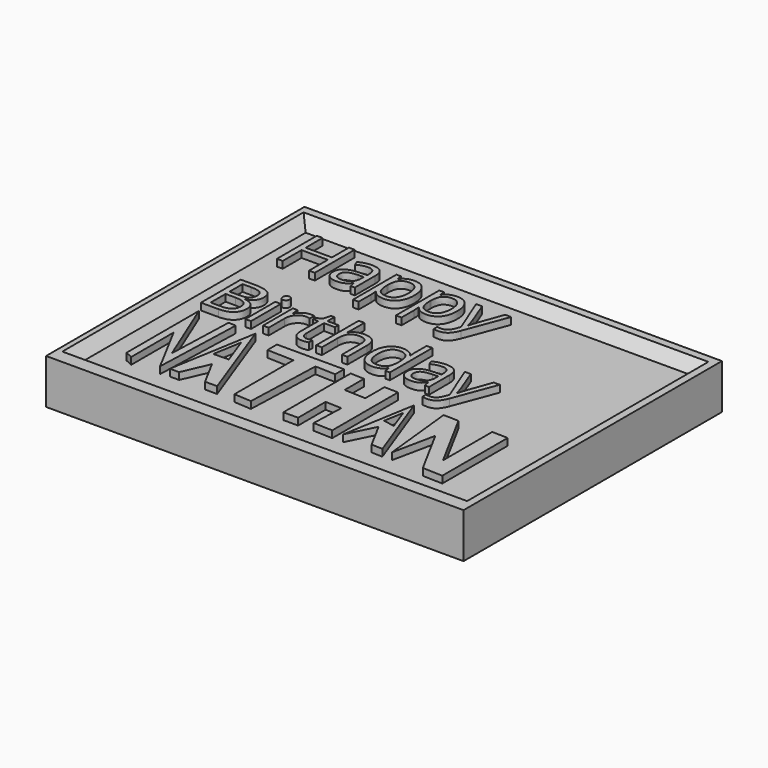
from build123d import *

# Parameters (mm, degrees)
F1_W         = 153.5131447017
F1_H         = 118.7682263553
F1_W_2       = 138.6890634894
F1_H_2       = 100.725505501
F2_DEPTH     = 16.51
F3_DEPTH     = 12.7
F0_TEXT_SIZE = 25.6912866866
F4_DEPTH     = 15.24
F5_T4_DEPTH  = 138.6890634894
F5_T9_DEPTH  = 100.725505501
F5_T14_DEPTH = 138.6890634894
F5_T19_DEPTH = 100.725505501
F5_T25_DEPTH = 113.7896550799
F5_T30_DEPTH = 151.7532130683
F5_T38_DEPTH = 151.7532130683
F5_T43_DEPTH = 113.7896550799
F5_T51_DEPTH = 113.7896550799
F5_T56_DEPTH = 151.7532130683
F5_T64_DEPTH = 113.7896550799
F5_T69_DEPTH = 151.7532130683


# Not quite as in the source:
# - a fillet or chamfer that OpenCascade refuses, or shapes differently, is made with other operations: its cross-section is extruded or revolved along the edge and cut away or added
# - Text() gives the source's letters only with a copy of the font that has no kerning and outlines rounded to 1/6400 em; it was checked with that copy


with BuildPart() as f2:
    # F1 (on Top) → F2 (new body)
    with BuildSketch(Plane.XY):
        with Locations((-23.7906444818, -12.9123348743)):
            Rectangle(F1_W, F1_H)
        with Locations((-24.1845287383, -11.8035394698)):
            Rectangle(F1_W_2, F1_H_2, mode=Mode.SUBTRACT)
    extrude(amount=F2_DEPTH)

    # F1 (on Top) → F3 (join)
    with BuildSketch(Plane.XY):
        with Locations((-24.1845287383, -11.8035394698)):
            Rectangle(F1_W_2, F1_H_2)
    extrude(amount=F3_DEPTH)

    # F0 (on Top) → F4 (join)
    with BuildSketch(Plane.XY):
        Polygon((-85.3031873703, -21.0467930883), (-85.3031873703, -54.3782301247), (-82.5872942805, -55.6127279997), (-82.5872942805, -36.1076667905), (-72.49553914, -54.9944023292), (-71.3395271598, -21.6351880797), (-74.0692615509, -21.5405933559), (-74.9334096909, -46.4774481952), align=None)
        Polygon((-63.8229250908, -22.0343936235), (-69.3781673908, -54.3782301247), (-65.9531280398, -54.3782301247), (-61.6957172751, -44.6236543357), (-56.4159415662, -54.3782301247), (-51.9717484713, -54.3782301247), align=None)
        Polygon((-59.7228327978, -39.3131503296), (-65.3510764241, -39.4346043468), (-63.5406248941, -28.8937593002), align=None, mode=Mode.SUBTRACT)
        Polygon((-44.9698902667, -28.1148646027), (-44.9698902667, -55.175434798), (-38.6008597223, -55.5698666259), (-37.6162595271, -27.157108435), (-30.1302243024, -27.4165254086), (-30.1302243024, -23.4010890126), (-54.7469718501, -23.4010890126), (-54.7469718501, -27.7760549605), align=None)
        Polygon((-26.9877053797, -24.2740083486), (-26.9877053797, -55.175434798), (-21.5674239871, -55.175434798), (-21.5674239871, -42.544283495), (-15.5946510085, -42.7512607057), (-16.0167792908, -54.9326810121), (-9.0115962201, -55.175434798), (-9.0115962201, -24.9731168782), (-14.0718441197, -24.7977618128), (-14.0718441197, -33.6245252917), (-21.92478826, -33.352393657), (-21.92478826, -24.4494559116), align=None)
        Polygon((-0.3970701119, -28.3770595024), (-4.9998471513, -55.175434798), (0, -45.1317872426), (5.3600473669, -55.0346678109), (9.4221818105, -55.175434798), align=None)
        Polygon((3.0691473118, -41.9747008738), (-1.1165549513, -41.2297546864), (0.1321939148, -33.9592654843), align=None, mode=Mode.SUBTRACT)
        Polygon((10.0144669414, -27.7569666505), (12.9211032763, -55.175434798), (16.226188811, -39.3131503296), (25.9121123405, -57.2082429175), (33.2773711625, -57.4634745717), (33.2773711625, -27.4220021975), (27.4817449731, -27.2211637348), (27.4817449731, -49.8912126499), (15.6062132016, -27.9507399696), align=None)
        with Locations((-90.5801325571, 18.2041097432)):
            Text('Happy', F0_TEXT_SIZE, font='Open Sans', text_align=(TextAlign.LEFT, TextAlign.BOTTOM))
        with Locations((-90.5801325571, -16.7360401505)):
            Text('Birthday', F0_TEXT_SIZE, font='Open Sans', text_align=(TextAlign.LEFT, TextAlign.BOTTOM))
    extrude(amount=F4_DEPTH)

    # F5: chamfer of 5.08 on 4 edges, made by hand


with BuildPart() as f5_tool2:
    # F5_s3 → F5_t4 (new body)
    with BuildSketch(Plane.YZ.offset(-93.529060483)):
        Polygon((43.6392132807, 16.51), (38.5592132807, 11.43), (38.5592132807, 16.51), align=None)
    extrude(amount=F5_T4_DEPTH)

    split(bisect_by=Plane.XY.offset(12.7), keep=Keep.TOP)


with BuildPart() as f2_1:
    add(f2.part)

    # F5_t1: cut F5_tool2
    add(f5_tool2.part, mode=Mode.SUBTRACT)


with BuildPart() as f5_tool7:
    # F5_s8 → F5_t9 (new body)
    with BuildSketch(Plane.XZ.offset(-38.5592132807)):
        Polygon((50.2400030065, 16.51), (45.1600030065, 11.43), (45.1600030065, 16.51), align=None)
    extrude(amount=F5_T9_DEPTH)

    split(bisect_by=Plane.XY.offset(12.7), keep=Keep.TOP)


with BuildPart() as f2_2:
    add(f2_1.part)

    # F5_t6: cut F5_tool7
    add(f5_tool7.part, mode=Mode.SUBTRACT)


with BuildPart() as f5_tool12:
    # F5_s13 → F5_t14 (new body)
    with BuildSketch(Plane.YZ.offset(45.1600030065)):
        Polygon((-67.2462922204, 16.51), (-62.1662922204, 11.43), (-62.1662922204, 16.51), align=None)
    extrude(amount=-F5_T14_DEPTH)

    split(bisect_by=Plane.XY.offset(12.7), keep=Keep.TOP)


with BuildPart() as f2_3:
    add(f2_2.part)

    # F5_t11: cut F5_tool12
    add(f5_tool12.part, mode=Mode.SUBTRACT)


with BuildPart() as f5_tool17:
    # F5_s18 → F5_t19 (new body)
    with BuildSketch(Plane.XZ.offset(62.1662922204)):
        Polygon((-98.609060483, 16.51), (-93.529060483, 11.43), (-93.529060483, 16.51), align=None)
    extrude(amount=-F5_T19_DEPTH)

    split(bisect_by=Plane.XY.offset(12.7), keep=Keep.TOP)


with BuildPart() as f2_4:
    add(f2_3.part)

    # F5_t16: cut F5_tool17
    add(f5_tool17.part, mode=Mode.SUBTRACT)


with BuildPart() as f5_tool23:
    # F5_s24 → F5_t25 (new body)
    with BuildSketch(Plane.XZ.offset(62.1662922204)):
        Polygon((-98.609060483, 16.51), (-93.529060483, 11.43), (-93.529060483, 16.51), align=None)
    extrude(amount=-F5_T25_DEPTH)

    split(bisect_by=Plane.XY.offset(12.7), keep=Keep.TOP)

    split(bisect_by=Plane.XZ.offset(-38.5592132807), keep=Keep.BOTTOM)


with BuildPart() as f5_tool28:
    # F5_s29 → F5_t30 (new body)
    with BuildSketch(Plane.YZ.offset(-106.5932100618)):
        Polygon((43.6392132807, 16.51), (38.5592132807, 11.43), (38.5592132807, 16.51), align=None)
    extrude(amount=F5_T30_DEPTH)

    split(bisect_by=Plane.YZ.offset(-93.529060483), keep=Keep.BOTTOM)

    split(bisect_by=Plane.XY.offset(12.7), keep=Keep.TOP)


with BuildPart() as f5_tool23_1:
    add(f5_tool23.part)

    # F5_t33: intersect F5_tool28
    add(f5_tool28.part, mode=Mode.INTERSECT)


with BuildPart() as f2_5:
    add(f2_4.part)

    # F5_t21: cut F5_tool23
    add(f5_tool23_1.part, mode=Mode.SUBTRACT)


with BuildPart() as f5_tool36:
    # F5_s37 → F5_t38 (new body)
    with BuildSketch(Plane.YZ.offset(-93.529060483)):
        Polygon((43.6392132807, 16.51), (38.5592132807, 11.43), (38.5592132807, 16.51), align=None)
    extrude(amount=F5_T38_DEPTH)

    split(bisect_by=Plane.XY.offset(12.7), keep=Keep.TOP)

    split(bisect_by=Plane.YZ.offset(45.1600030065), keep=Keep.TOP)


with BuildPart() as f5_tool41:
    # F5_s42 → F5_t43 (new body)
    with BuildSketch(Plane.XZ.offset(-51.6233628595)):
        Polygon((50.2400030065, 16.51), (45.1600030065, 11.43), (45.1600030065, 16.51), align=None)
    extrude(amount=F5_T43_DEPTH)

    split(bisect_by=Plane.XZ.offset(-38.5592132807), keep=Keep.BOTTOM)

    split(bisect_by=Plane.XY.offset(12.7), keep=Keep.TOP)


with BuildPart() as f5_tool36_1:
    add(f5_tool36.part)

    # F5_t46: intersect F5_tool41
    add(f5_tool41.part, mode=Mode.INTERSECT)


with BuildPart() as f2_6:
    add(f2_5.part)

    # F5_t34: cut F5_tool36
    add(f5_tool36_1.part, mode=Mode.SUBTRACT)


with BuildPart() as f5_tool49:
    # F5_s50 → F5_t51 (new body)
    with BuildSketch(Plane.XZ.offset(-38.5592132807)):
        Polygon((50.2400030065, 16.51), (45.1600030065, 11.43), (45.1600030065, 16.51), align=None)
    extrude(amount=F5_T51_DEPTH)

    split(bisect_by=Plane.XY.offset(12.7), keep=Keep.TOP)

    split(bisect_by=Plane.XZ.offset(62.1662922204), keep=Keep.TOP)


with BuildPart() as f5_tool54:
    # F5_s55 → F5_t56 (new body)
    with BuildSketch(Plane.YZ.offset(58.2241525853)):
        Polygon((-67.2462922204, 16.51), (-62.1662922204, 11.43), (-62.1662922204, 16.51), align=None)
    extrude(amount=-F5_T56_DEPTH)

    split(bisect_by=Plane.YZ.offset(45.1600030065), keep=Keep.TOP)

    split(bisect_by=Plane.XY.offset(12.7), keep=Keep.TOP)


with BuildPart() as f5_tool49_1:
    add(f5_tool49.part)

    # F5_t59: intersect F5_tool54
    add(f5_tool54.part, mode=Mode.INTERSECT)


with BuildPart() as f2_7:
    add(f2_6.part)

    # F5_t47: cut F5_tool49
    add(f5_tool49_1.part, mode=Mode.SUBTRACT)


with BuildPart() as f5_tool62:
    # F5_s63 → F5_t64 (new body)
    with BuildSketch(Plane.XZ.offset(75.2304417992)):
        Polygon((-98.609060483, 16.51), (-93.529060483, 11.43), (-93.529060483, 16.51), align=None)
    extrude(amount=-F5_T64_DEPTH)

    split(bisect_by=Plane.XY.offset(12.7), keep=Keep.TOP)

    split(bisect_by=Plane.XZ.offset(62.1662922204), keep=Keep.TOP)


with BuildPart() as f5_tool67:
    # F5_s68 → F5_t69 (new body)
    with BuildSketch(Plane.YZ.offset(45.1600030065)):
        Polygon((-67.2462922204, 16.51), (-62.1662922204, 11.43), (-62.1662922204, 16.51), align=None)
    extrude(amount=-F5_T69_DEPTH)

    split(bisect_by=Plane.YZ.offset(-93.529060483), keep=Keep.BOTTOM)

    split(bisect_by=Plane.XY.offset(12.7), keep=Keep.TOP)


with BuildPart() as f5_tool62_1:
    add(f5_tool62.part)

    # F5_t72: intersect F5_tool67
    add(f5_tool67.part, mode=Mode.INTERSECT)


with BuildPart() as f2_8:
    add(f2_7.part)

    # F5_t60: cut F5_tool62
    add(f5_tool62_1.part, mode=Mode.SUBTRACT)


solid = f2_8.part
